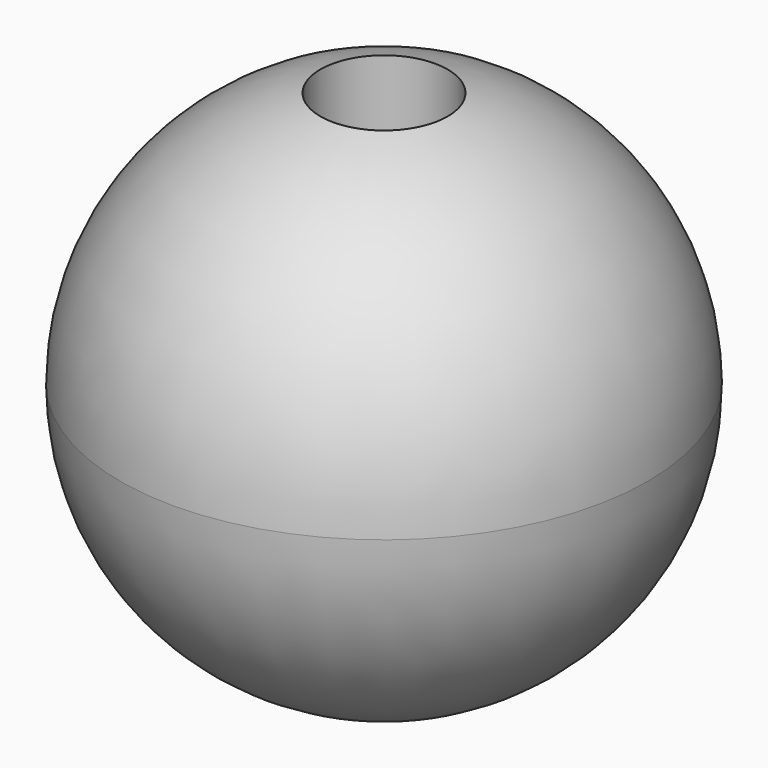
from build123d import *

# Parameters (mm, degrees)
F0_R          = 26.9875
F1_DEPTH      = 26.9875
F1_DEPTH_BACK = 26.9875
F3_R          = 26.98749
F2_R          = 6.5054455224
F4_DEPTH      = 31.75


# Not quite as in the source:
# - a fillet or chamfer is up to 0.001 mm smaller than in the source, because OpenCascade refuses the exact size


with BuildPart() as f1:
    # F0 (on Top) → F1 (new body, two sides)
    with BuildSketch(Plane.XY) as f1_sk:
        Circle(F0_R)
    extrude(amount=F1_DEPTH)
    extrude(f1_sk.sketch, amount=-F1_DEPTH_BACK)

    # F3 (radius 26.9875 in the source; OpenCascade refuses exactly that, so slightly less here)
    f3_edges = [f1.edges().sort_by_distance(p)[0] for p in [
        (-26.9875, 0, 26.9875),
        (-26.9875, 0, -26.9875),
    ]]
    fillet(f3_edges, radius=F3_R)

    # F2 (on face) → F4 (cut)
    with BuildSketch(Plane.XY.offset(26.9875)):
        Circle(F2_R)
    extrude(amount=-F4_DEPTH, mode=Mode.SUBTRACT)


solid = f1.part
